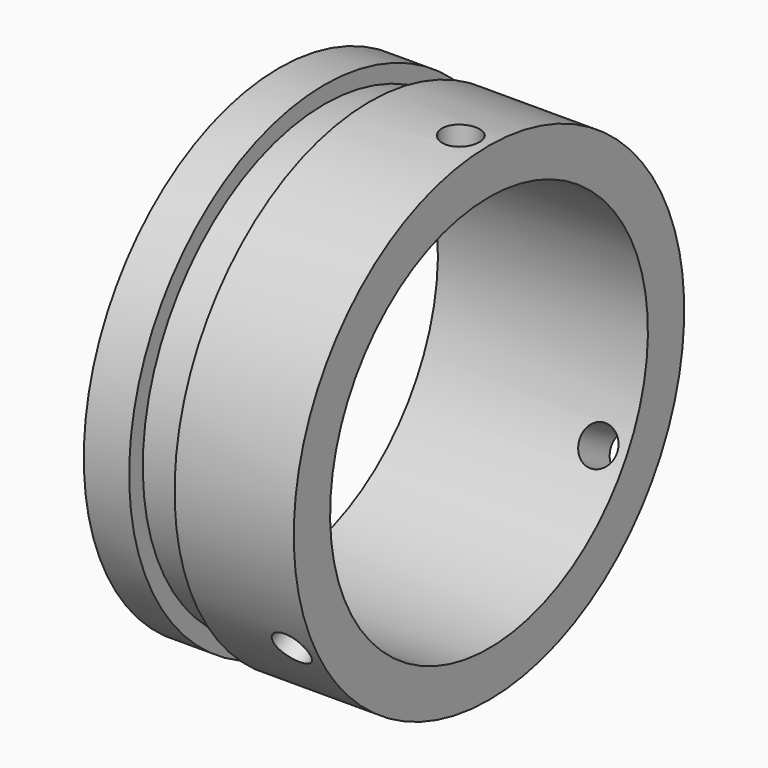
from build123d import *

# Parameters (mm, degrees)
F5_D            = 6.6
F5_DEPTH        = 15
F5_START        = 0.126815
F5_TIP          = 1.9828400428
F5_COPIES_COUNT = 3


# Not quite as in the source:
# - a pattern or mirror of a feature is missing from the dataset's text; its kind, count and spacing are read off the source's solid


with BuildPart() as f1:
    # F0 (on Front) → F1 (revolve)
    with BuildSketch(Plane.XZ):
        Polygon((0, 43), (0, 35), (37, 35), (37, 43), (16, 43), (16, 40), (8, 40), (8, 43), align=None)
    revolve(axis=Axis((12.3033272102, 0, 0), (1, 0, 0)))

    # F5
    # its depths count from where the whole tool has entered the part; down to there all is cleared
    with Locations(Plane.XY.offset(43).offset(-F5_START)):
        with Locations((32.0342332125, 0)):
            f5 = Hole(F5_D / 2, depth=F5_DEPTH)
            with Locations((0, 0, -(F5_DEPTH + F5_TIP / 2))):  # 118° drill point
                Cone(0, F5_D / 2, F5_TIP, mode=Mode.SUBTRACT)

    # F5_copies: F5 ×3 about axis
    f5_copies_axis = Axis((0, 0, 0), (1, 0, 0))
    for i in range(1, F5_COPIES_COUNT):
        add(f5.rotate(f5_copies_axis, i * 360 / F5_COPIES_COUNT), mode=Mode.SUBTRACT)


solid = f1.part
